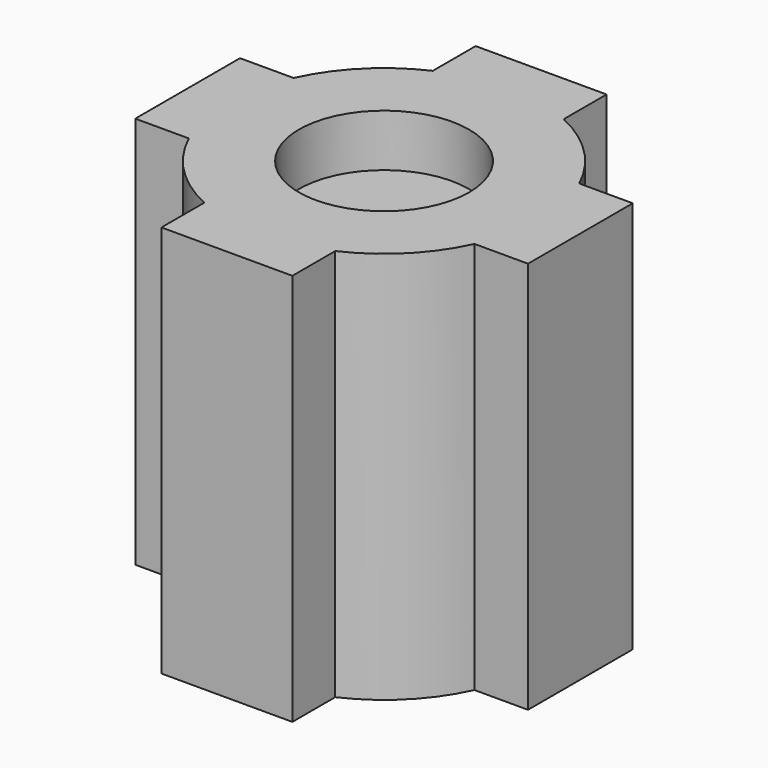
from build123d import *

# Parameters (mm, degrees)
F0_W     = 5
F0_H     = 5
F1_DEPTH = 3
F5_DEPTH = 5
F7_DEPTH = 7
F8_R     = 3.25
F9_DEPTH = 2


with BuildPart() as f1:
    # F0 (on Top) → F1 (new body)
    with BuildSketch(Plane.XY):
        with BuildLine():
            Line((2.5, 2.5), (5.4543560573, 2.5))
            ThreePointArc((5.4543560573, 2.5), (4.2426406871, 4.2426406871), (2.5, 5.4543560573))
            Line((2.5, 5.4543560573), (2.5, 2.5))
        make_face()
        with BuildLine():
            Line((2.5, -7.5), (2.5, -5.4543560573))
            ThreePointArc((2.5, -5.4543560573), (0, -6), (-2.5, -5.4543560573))
            Line((-2.5, -5.4543560573), (-2.5, -7.5))
            Line((-2.5, -7.5), (2.5, -7.5))
        make_face()
        with BuildLine():
            ThreePointArc((-5.4543560573, -2.5), (-4.2426406871, -4.2426406871), (-2.5, -5.4543560573))
            Line((-2.5, -5.4543560573), (-2.5, -2.5))
            Line((-2.5, -2.5), (-5.4543560573, -2.5))
        make_face()
        with BuildLine():
            ThreePointArc((-5.4543560573, -2.5), (-6, 0), (-5.4543560573, 2.5))
            Line((-5.4543560573, 2.5), (-7.5, 2.5))
            Line((-7.5, 2.5), (-7.5, -2.5))
            Line((-7.5, -2.5), (-5.4543560573, -2.5))
        make_face()
        with BuildLine():
            ThreePointArc((2.5, -5.4543560573), (4.2426406871, -4.2426406871), (5.4543560573, -2.5))
            Line((5.4543560573, -2.5), (2.5, -2.5))
            Line((2.5, -2.5), (2.5, -5.4543560573))
        make_face()
        with BuildLine():
            Line((-2.5, 2.5), (-2.5, 5.4543560573))
            ThreePointArc((-2.5, 5.4543560573), (-4.2426406871, 4.2426406871), (-5.4543560573, 2.5))
            Line((-5.4543560573, 2.5), (-2.5, 2.5))
        make_face()
        with BuildLine():
            ThreePointArc((5.4543560573, -2.5), (5.8620020617, -1.2794263668), (6, 0))
            ThreePointArc((6, 0), (5.8620020617, 1.2794263668), (5.4543560573, 2.5))
            Line((5.4543560573, 2.5), (2.5, 2.5))
            Line((2.5, 2.5), (2.5, -2.5))
            Line((2.5, -2.5), (5.4543560573, -2.5))
        make_face()
        Rectangle(F0_W, F0_H)
        with BuildLine():
            Line((-2.5, -2.5), (-2.5, 2.5))
            Line((-2.5, 2.5), (-5.4543560573, 2.5))
            ThreePointArc((-5.4543560573, 2.5), (-6, 0), (-5.4543560573, -2.5))
            Line((-5.4543560573, -2.5), (-2.5, -2.5))
        make_face()
        with BuildLine():
            Line((2.5, 2.5), (2.5, 5.4543560573))
            ThreePointArc((2.5, 5.4543560573), (0, 6), (-2.5, 5.4543560573))
            Line((-2.5, 5.4543560573), (-2.5, 2.5))
            Line((-2.5, 2.5), (2.5, 2.5))
        make_face()
        with BuildLine():
            ThreePointArc((-2.5, 5.4543560573), (0, 6), (2.5, 5.4543560573))
            Line((2.5, 5.4543560573), (2.5, 7.5))
            Line((2.5, 7.5), (-2.5, 7.5))
            Line((-2.5, 7.5), (-2.5, 5.4543560573))
        make_face()
        with BuildLine():
            ThreePointArc((5.4543560573, 2.5), (5.8620020617, 1.2794263668), (6, 0))
            ThreePointArc((6, 0), (5.8620020617, -1.2794263668), (5.4543560573, -2.5))
            Line((5.4543560573, -2.5), (7.5, -2.5))
            Line((7.5, -2.5), (7.5, 2.5))
            Line((7.5, 2.5), (5.4543560573, 2.5))
        make_face()
        with BuildLine():
            ThreePointArc((-2.5, -5.4543560573), (0, -6), (2.5, -5.4543560573))
            Line((2.5, -5.4543560573), (2.5, -2.5))
            Line((2.5, -2.5), (-2.5, -2.5))
            Line((-2.5, -2.5), (-2.5, -5.4543560573))
        make_face()
    extrude(amount=F1_DEPTH)

    # F5 (add): a face of the model
    f5_faces = [f1.faces().sort_by_distance(p)[0] for p in [
        (0, 0, 0),
    ]]
    extrude(f5_faces, amount=F5_DEPTH)


with BuildPart() as f4:
    # F3 (on Right) → F4 (revolve)
    with BuildSketch(Plane.YZ):
        with BuildLine():
            Line((0, -12), (0, 0))
            ThreePointArc((0, 0), (-6, -6), (0, -12))
        make_face()
    revolve(axis=Axis((0, 0, -6), (0, 0, -1)))


with BuildPart() as f1_1:
    add(f1.part)

    # F6: cut F4
    add(f4.part, mode=Mode.SUBTRACT)

    # F2 (on face) → F7 (join)
    with BuildSketch(Plane.XY.offset(3)):
        with BuildLine():
            ThreePointArc((-2.5, 5.4543560573), (-4.2426406871, 4.2426406871), (-5.4543560573, 2.5))
            Line((-5.4543560573, 2.5), (-7.5, 2.5))
            Line((-7.5, 2.5), (-7.5, -2.5))
            Line((-7.5, -2.5), (-5.4543560573, -2.5))
            ThreePointArc((-5.4543560573, -2.5), (-4.2426406871, -4.2426406871), (-2.5, -5.4543560573))
            Line((-2.5, -5.4543560573), (-2.5, -7.5))
            Line((-2.5, -7.5), (2.5, -7.5))
            Line((2.5, -7.5), (2.5, -5.4543560573))
            ThreePointArc((2.5, -5.4543560573), (4.2426406871, -4.2426406871), (5.4543560573, -2.5))
            Line((5.4543560573, -2.5), (7.5, -2.5))
            Line((7.5, -2.5), (7.5, 2.5))
            Line((7.5, 2.5), (5.4543560573, 2.5))
            ThreePointArc((5.4543560573, 2.5), (4.2426406871, 4.2426406871), (2.5, 5.4543560573))
            Line((2.5, 5.4543560573), (2.5, 7.5))
            Line((2.5, 7.5), (-2.5, 7.5))
            Line((-2.5, 7.5), (-2.5, 5.4543560573))
        make_face()
    extrude(amount=F7_DEPTH)

    # F8 (on face) → F9 (cut)
    with BuildSketch(Plane.XY.offset(10)):
        Circle(F8_R)
    extrude(amount=-F9_DEPTH, mode=Mode.SUBTRACT)


solid = f1_1.part
